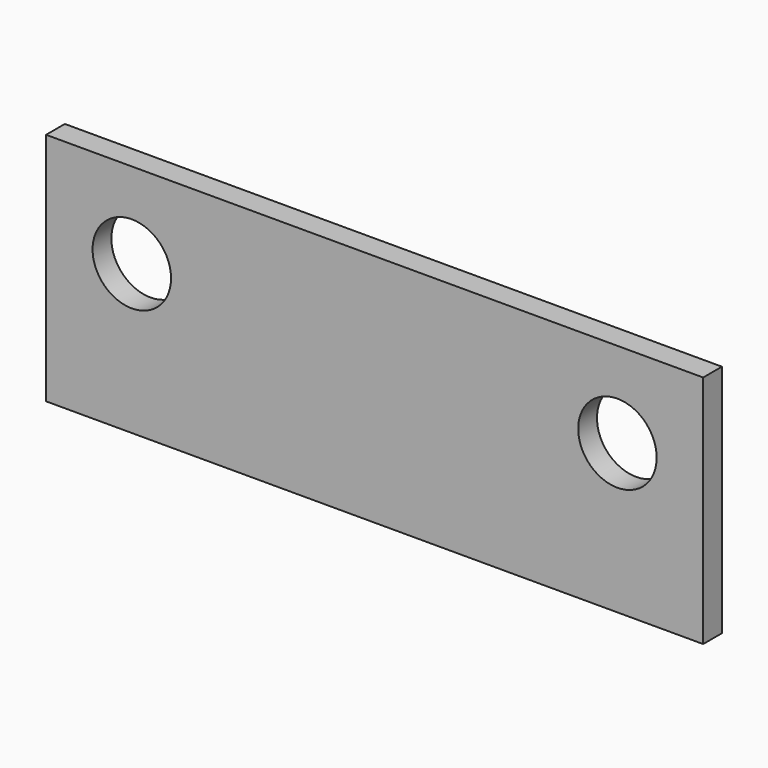
from build123d import *

# Parameters (mm, degrees)
F0_R     = 21.2328125
F1_DEPTH = 12.7
F2_DEPTH = 385


# Not quite as in the source:
# - an extrude ends at something that could not be found from the text; its depth is read off the source's solid


with BuildPart() as f1:
    # F0 (on Front) → F1 (new body)
    with BuildSketch(Plane.XZ):
        Polygon((177.8, 17.1069), (177.8, 63.5), (131.4069, 63.5), (-131.4069, 63.5), (-177.8, 63.5), (-177.8, 17.1069), (-177.8, -63.5), (177.8, -63.5), align=None)
        with Locations((-131.4069, 17.1069)):
            Circle(F0_R, mode=Mode.SUBTRACT)
        with Locations((131.4069, 17.1069)):
            Circle(F0_R, mode=Mode.SUBTRACT)
    extrude(amount=F1_DEPTH)

    # F0 (on Front) → F2 (cut, through all)
    with BuildSketch(Plane.XZ):
        Polygon((177.8, 17.1069), (177.8, 63.5), (131.4069, 63.5), (-131.4069, 63.5), (-177.8, 63.5), (-177.8, 17.1069), (-177.8, -63.5), (177.8, -63.5), align=None)
        with Locations((-131.4069, 17.1069)):
            Circle(F0_R, mode=Mode.SUBTRACT)
        with Locations((131.4069, 17.1069)):
            Circle(F0_R, mode=Mode.SUBTRACT)
    extrude(amount=-F2_DEPTH, mode=Mode.SUBTRACT)


solid = f1.part
